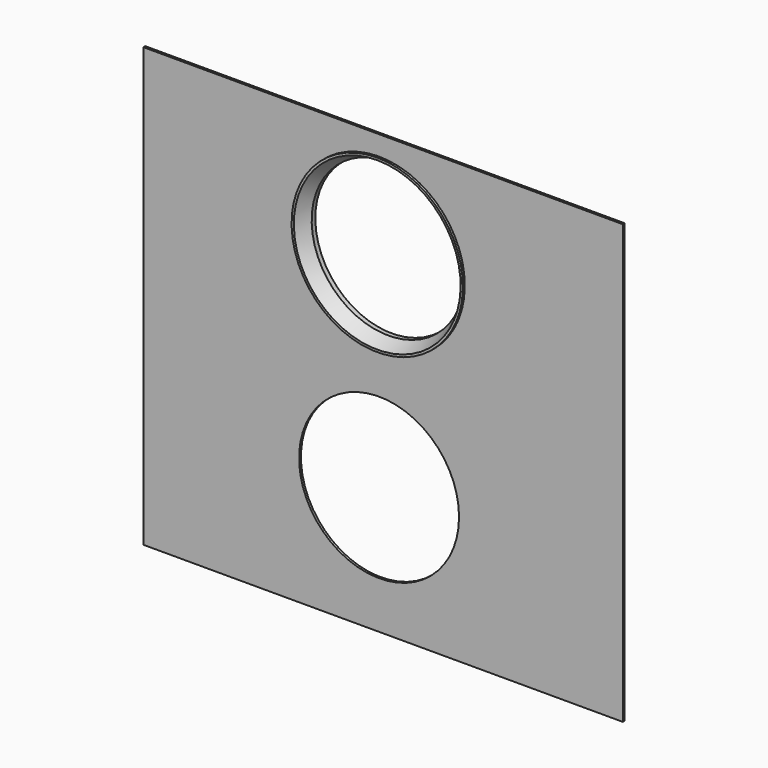
from build123d import *

# Parameters (mm, degrees)
F1_W     = 209.9018618464
F1_H     = 191.7395107448
F1_R     = 35
F1_R_2   = 37.5
F2_DEPTH = 1
F5_W     = 80
F5_H     = 80
F5_R     = 1.1
F5_R_2   = 37.5
F6_DEPTH = 1
F7_DEPTH = 2


with BuildPart() as f2:
    # F1 (on offset) → F2 (new body)
    with BuildSketch(Plane.XZ.offset(5)):
        with Locations((1.7582438886, -49.7746858746)):
            Rectangle(F1_W, F1_H)
        with Locations((0, -90)):
            Circle(F1_R, mode=Mode.SUBTRACT)
        Circle(F1_R_2, mode=Mode.SUBTRACT)
    extrude(amount=-F2_DEPTH)


with BuildPart() as f4:
    # F3 (on Right) → F4 (revolve)
    with BuildSketch(Plane.YZ):
        Polygon((0, 37.5), (-6, 37.5), (-6, 36.5), (0, 33.5), align=None)
    revolve(axis=Axis((0, 1.602868408, 0), (0, -1, 0)))

    # F7 (add): a face of the model
    f7_faces = [f4.faces().sort_by_distance(p)[0] for p in [
        (0, 0, -34.5606601718),
    ]]
    extrude(f7_faces, amount=F7_DEPTH)


with BuildPart() as f6:
    # F5 (on Front) → F6 (new body)
    with BuildSketch(Plane.XZ):
        Rectangle(F5_W, F5_H)
        with Locations((-30, -30)):
            Circle(F5_R, mode=Mode.SUBTRACT)
        with Locations((30, -30)):
            Circle(F5_R, mode=Mode.SUBTRACT)
        with Locations((-30, 30)):
            Circle(F5_R, mode=Mode.SUBTRACT)
        Circle(F5_R_2, mode=Mode.SUBTRACT)
        with Locations((30, 30)):
            Circle(F5_R, mode=Mode.SUBTRACT)
    extrude(amount=F6_DEPTH)


solid = Compound([f2.part, f4.part, f6.part])
